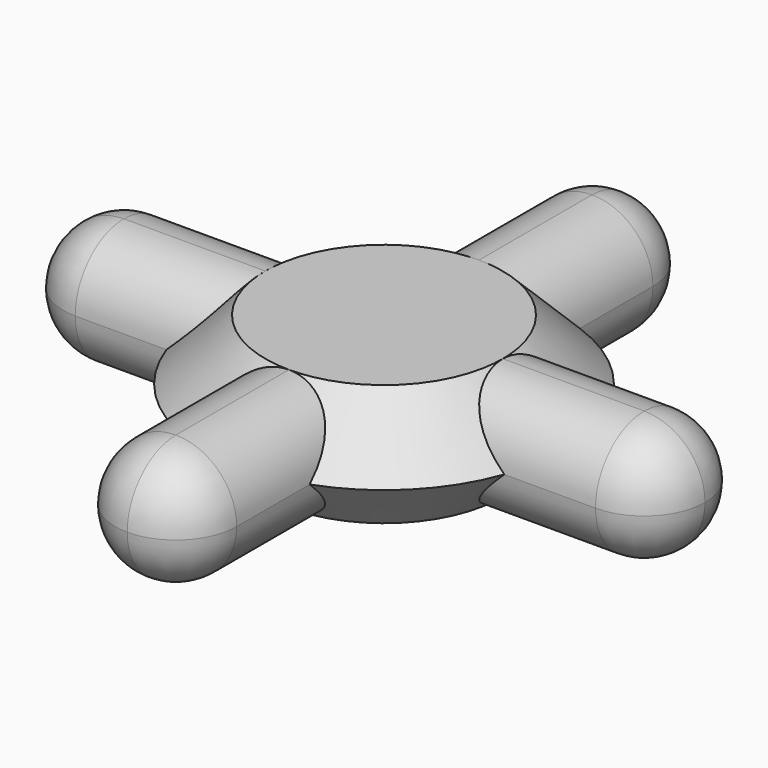
from build123d import *

# Parameters (mm, degrees)
F0_R     = 6.35
F0_R_2   = 3.175
F2_DEPTH = 10.16
F3_SIZE  = 5.07999
F4_R     = 5.07999


# Not quite as in the source:
# - a fillet or chamfer is up to 0.001 mm smaller than in the source, because OpenCascade refuses the exact size


with BuildPart() as f2:
    # F0 (on Top) → F2 (new body)
    with BuildSketch(Plane.XY):
        Circle(F0_R)
        Circle(F0_R_2, mode=Mode.SUBTRACT)
        Circle(F0_R_2)
    extrude(amount=F2_DEPTH)


with BuildPart() as f2b:
    # F1 (on Top) → F2, piece 2 (new body)
    with BuildSketch(Plane.XY):
        with BuildLine():
            ThreePointArc((-5.08, 14.1135962816), (0, 15), (5.08, 14.1135962816))
            Line((5.08, 14.1135962816), (5.08, 21.7335962816))
            ThreePointArc((5.08, 21.7335962816), (3.5921024484, 25.32569873), (0, 26.8135962816))
            ThreePointArc((0, 26.8135962816), (-3.5921024484, 25.32569873), (-5.08, 21.7335962816))
            Line((-5.08, 21.7335962816), (-5.08, 14.1135962816))
        make_face()
        with BuildLine():
            ThreePointArc((-14.1135962816, -5.08), (-15, 0), (-14.1135962816, 5.08))
            Line((-14.1135962816, 5.08), (-21.7335962816, 5.08))
            ThreePointArc((-21.7335962816, 5.08), (-25.32569873, 3.5921024484), (-26.8135962816, 0))
            ThreePointArc((-26.8135962816, 0), (-25.32569873, -3.5921024484), (-21.7335962816, -5.08))
            Line((-21.7335962816, -5.08), (-14.1135962816, -5.08))
        make_face()
        with BuildLine():
            Line((5.08, -21.7335962816), (5.08, -14.1135962816))
            ThreePointArc((5.08, -14.1135962816), (0, -15), (-5.08, -14.1135962816))
            Line((-5.08, -14.1135962816), (-5.08, -21.7335962816))
            ThreePointArc((-5.08, -21.7335962816), (-3.5921024484, -25.32569873), (0, -26.8135962816))
            ThreePointArc((0, -26.8135962816), (3.5921024484, -25.32569873), (5.08, -21.7335962816))
        make_face()
        with BuildLine():
            ThreePointArc((14.1135962816, 5.08), (14.7767375328, 2.5783769872), (15, 0))
            ThreePointArc((15, 0), (14.7767375328, -2.5783769872), (14.1135962816, -5.08))
            Line((14.1135962816, -5.08), (21.7335962816, -5.08))
            ThreePointArc((21.7335962816, -5.08), (25.32569873, -3.5921024484), (26.8135962816, 0))
            ThreePointArc((26.8135962816, 0), (25.32569873, 3.5921024484), (21.7335962816, 5.08))
            Line((21.7335962816, 5.08), (14.1135962816, 5.08))
        make_face()
        with BuildLine():
            ThreePointArc((14.1135962816, -5.08), (14.7767375328, -2.5783769872), (15, 0))
            ThreePointArc((15, 0), (14.7767375328, 2.5783769872), (14.1135962816, 5.08))
            ThreePointArc((14.1135962816, 5.08), (10.6066017178, 10.6066017178), (5.08, 14.1135962816))
            ThreePointArc((5.08, 14.1135962816), (0, 15), (-5.08, 14.1135962816))
            ThreePointArc((-5.08, 14.1135962816), (-10.6066017178, 10.6066017178), (-14.1135962816, 5.08))
            ThreePointArc((-14.1135962816, 5.08), (-15, 0), (-14.1135962816, -5.08))
            ThreePointArc((-14.1135962816, -5.08), (-10.6066017178, -10.6066017178), (-5.08, -14.1135962816))
            ThreePointArc((-5.08, -14.1135962816), (0, -15), (5.08, -14.1135962816))
            ThreePointArc((5.08, -14.1135962816), (10.6066017178, -10.6066017178), (14.1135962816, -5.08))
        make_face()
    extrude(amount=F2_DEPTH)

    # F3 (size 5.08 in the source; OpenCascade refuses exactly that, so slightly less here)
    f3_edges = [f2b.edges().sort_by_distance(p)[0] for p in [
        (-10.606602, 10.606602, 10.16),
        (-10.606602, 10.606602, 0),
        (-10.606602, -10.606602, 0),
        (-10.606602, -10.606602, 10.16),
        (10.606602, -10.606602, 0),
        (10.606602, -10.606602, 10.16),
        (10.606602, 10.606602, 0),
        (10.606602, 10.606602, 10.16),
    ]]
    chamfer(f3_edges, length=F3_SIZE)

    # F4 (radius 5.08 in the source; OpenCascade refuses exactly that, so slightly less here)
    f4_edges = [f2b.edges().sort_by_distance(p)[0] for p in [
        (-5.08, 17.923596, 10.16),
        (-5.08, 17.923596, 0),
        (-17.923596, -5.08, 10.16),
        (-17.923596, -5.08, 0),
        (17.923596, 5.08, 10.16),
        (17.923596, 5.08, 0),
        (-5.08, -17.923596, 10.16),
        (-5.08, -17.923596, 0),
    ]]
    fillet(f4_edges, radius=F4_R)


solid = Compound([f2.part, f2b.part])
